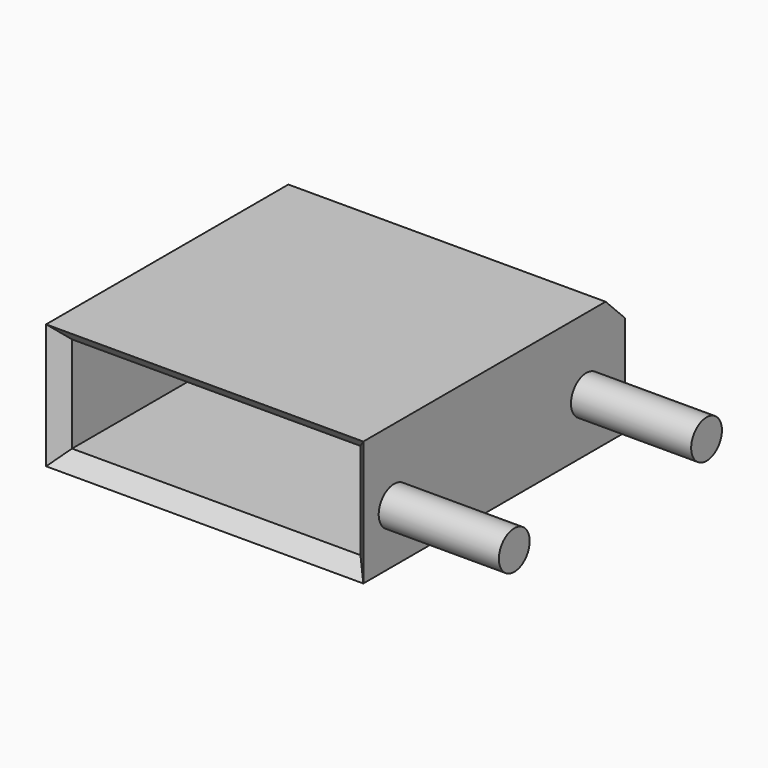
from build123d import *

# Parameters (mm, degrees)
F0_W         = 66
F0_H         = 26
F0_W_2       = 60
F0_H_2       = 20
F1_DEPTH     = 70
F2_R         = 4
F3_DEPTH     = 25
F4_T1_DEPTH  = 60
F4_T3_DEPTH  = 20
F4_T9_DEPTH  = 72.8584149398
F4_T15_DEPTH = 32.8584149398
F4_T24_DEPTH = 72.8584149398
F4_T30_DEPTH = 32.8584149398
F4_T39_DEPTH = 72.8584149398
F4_T45_DEPTH = 32.8584149398
F4_T54_DEPTH = 32.8584149398
F4_T60_DEPTH = 72.8584149398
F5_T1_DEPTH  = 91.7168298797


# Not quite as in the source:
# - a fillet or chamfer that OpenCascade refuses, or shapes differently, is made with other operations: its cross-section is extruded or revolved along the edge and cut away or added


with BuildPart() as f1:
    # F0 (on Front) → F1 (new body)
    with BuildSketch(Plane.XZ):
        with Locations((1.3007868016, 6.4724322181)):
            Rectangle(F0_W, F0_H)
        with Locations((1.3007868016, 6.4724322181)):
            Rectangle(F0_W_2, F0_H_2, mode=Mode.SUBTRACT)
    extrude(amount=F1_DEPTH)

    # F2 (on face) → F3 (join)
    with BuildSketch(Plane.YZ.offset(34.3007868016)):
        with Locations((-60, 4.4724322181)):
            Circle(F2_R)
        with Locations((-10, 4.4724322181)):
            Circle(F2_R)
    extrude(amount=F3_DEPTH)

    # F4: chamfer of 5 on 4 edges, made by hand

    # F4_s2 → F4_t1 (cut)
    with BuildSketch(Plane.YZ.offset(-28.6992131984)):
        Polygon((-70, 21.4724322181), (-65, 16.4724322181), (-70, 16.4724322181), align=None)
        Polygon((-70, -8.5275677819), (-65, -3.5275677819), (-70, -3.5275677819), align=None)
    extrude(amount=F4_T1_DEPTH, mode=Mode.SUBTRACT)

    # F4_s4 → F4_t3 (cut)
    with BuildSketch(Plane.XY.offset(-3.5275677819)):
        Polygon((-33.6992131984, -70), (-28.6992131984, -65), (-28.6992131984, -70), align=None)
        Polygon((36.3007868016, -70), (31.3007868016, -65), (31.3007868016, -70), align=None)
    extrude(amount=F4_T3_DEPTH, mode=Mode.SUBTRACT)


with BuildPart() as f4_tool7:
    # F4_s8 → F4_t9 (new body)
    with BuildSketch(Plane.YZ.offset(-41.5576281383)):
        Polygon((-70, 21.4724322181), (-65, 16.4724322181), (-70, 16.4724322181), align=None)
    extrude(amount=F4_T9_DEPTH)

    split(bisect_by=Plane.YZ.offset(-31.6992131984), keep=Keep.TOP)

    split(bisect_by=Plane.XY.offset(19.4724322181), keep=Keep.BOTTOM)

    split(bisect_by=Plane.YZ.offset(-28.6992131984), keep=Keep.BOTTOM)


with BuildPart() as f4_tool13:
    # F4_s14 → F4_t15 (new body)
    with BuildSketch(Plane.XY.offset(-3.5275677819)):
        Polygon((-33.6992131984, -70), (-28.6992131984, -65), (-28.6992131984, -70), align=None)
    extrude(amount=F4_T15_DEPTH)

    split(bisect_by=Plane.YZ.offset(-31.6992131984), keep=Keep.TOP)

    split(bisect_by=Plane.XY.offset(19.4724322181), keep=Keep.BOTTOM)

    split(bisect_by=Plane.XY.offset(16.4724322181), keep=Keep.TOP)


with BuildPart() as f4_tool7_1:
    add(f4_tool7.part)

    # F4_t19: intersect F4_tool13
    add(f4_tool13.part, mode=Mode.INTERSECT)


with BuildPart() as f1_1:
    add(f1.part)

    # F4_t5: cut F4_tool7
    add(f4_tool7_1.part, mode=Mode.SUBTRACT)


with BuildPart() as f4_tool22:
    # F4_s23 → F4_t24 (new body)
    with BuildSketch(Plane.YZ.offset(-28.6992131984)):
        Polygon((-70, 21.4724322181), (-65, 16.4724322181), (-70, 16.4724322181), align=None)
    extrude(amount=F4_T24_DEPTH)

    split(bisect_by=Plane.YZ.offset(34.3007868016), keep=Keep.BOTTOM)

    split(bisect_by=Plane.XY.offset(19.4724322181), keep=Keep.BOTTOM)

    split(bisect_by=Plane.YZ.offset(31.3007868016), keep=Keep.TOP)


with BuildPart() as f4_tool28:
    # F4_s29 → F4_t30 (new body)
    with BuildSketch(Plane.XY.offset(29.3308471579)):
        Polygon((36.3007868016, -70), (31.3007868016, -65), (31.3007868016, -70), align=None)
    extrude(amount=-F4_T30_DEPTH)

    split(bisect_by=Plane.YZ.offset(34.3007868016), keep=Keep.BOTTOM)

    split(bisect_by=Plane.XY.offset(19.4724322181), keep=Keep.BOTTOM)

    split(bisect_by=Plane.XY.offset(16.4724322181), keep=Keep.TOP)


with BuildPart() as f4_tool22_1:
    add(f4_tool22.part)

    # F4_t34: intersect F4_tool28
    add(f4_tool28.part, mode=Mode.INTERSECT)


with BuildPart() as f1_2:
    add(f1_1.part)

    # F4_t20: cut F4_tool22
    add(f4_tool22_1.part, mode=Mode.SUBTRACT)


with BuildPart() as f4_tool37:
    # F4_s38 → F4_t39 (new body)
    with BuildSketch(Plane.YZ.offset(31.3007868016)):
        Polygon((-70, -8.5275677819), (-65, -3.5275677819), (-70, -3.5275677819), align=None)
    extrude(amount=-F4_T39_DEPTH)

    split(bisect_by=Plane.XY.offset(-6.5275677819), keep=Keep.TOP)

    split(bisect_by=Plane.YZ.offset(-31.6992131984), keep=Keep.TOP)

    split(bisect_by=Plane.YZ.offset(-28.6992131984), keep=Keep.BOTTOM)


with BuildPart() as f4_tool43:
    # F4_s44 → F4_t45 (new body)
    with BuildSketch(Plane.XY.offset(-16.3859827218)):
        Polygon((-33.6992131984, -70), (-28.6992131984, -65), (-28.6992131984, -70), align=None)
    extrude(amount=F4_T45_DEPTH)

    split(bisect_by=Plane.XY.offset(-6.5275677819), keep=Keep.TOP)

    split(bisect_by=Plane.YZ.offset(-31.6992131984), keep=Keep.TOP)

    split(bisect_by=Plane.XY.offset(-3.5275677819), keep=Keep.BOTTOM)


with BuildPart() as f4_tool37_1:
    add(f4_tool37.part)

    # F4_t49: intersect F4_tool43
    add(f4_tool43.part, mode=Mode.INTERSECT)


with BuildPart() as f1_3:
    add(f1_2.part)

    # F4_t35: cut F4_tool37
    add(f4_tool37_1.part, mode=Mode.SUBTRACT)


with BuildPart() as f4_tool52:
    # F4_s53 → F4_t54 (new body)
    with BuildSketch(Plane.XY.offset(16.4724322181)):
        Polygon((36.3007868016, -70), (31.3007868016, -65), (31.3007868016, -70), align=None)
    extrude(amount=-F4_T54_DEPTH)

    split(bisect_by=Plane.XY.offset(-6.5275677819), keep=Keep.TOP)

    split(bisect_by=Plane.YZ.offset(34.3007868016), keep=Keep.BOTTOM)

    split(bisect_by=Plane.XY.offset(-3.5275677819), keep=Keep.BOTTOM)


with BuildPart() as f4_tool58:
    # F4_s59 → F4_t60 (new body)
    with BuildSketch(Plane.YZ.offset(44.1592017414)):
        Polygon((-70, -8.5275677819), (-65, -3.5275677819), (-70, -3.5275677819), align=None)
    extrude(amount=-F4_T60_DEPTH)

    split(bisect_by=Plane.XY.offset(-6.5275677819), keep=Keep.TOP)

    split(bisect_by=Plane.YZ.offset(34.3007868016), keep=Keep.BOTTOM)

    split(bisect_by=Plane.YZ.offset(31.3007868016), keep=Keep.TOP)


with BuildPart() as f4_tool52_1:
    add(f4_tool52.part)

    # F4_t64: intersect F4_tool58
    add(f4_tool58.part, mode=Mode.INTERSECT)


with BuildPart() as f1_4:
    add(f1_3.part)

    # F4_t50: cut F4_tool52
    add(f4_tool52_1.part, mode=Mode.SUBTRACT)

    # F5: chamfer of 5 on 1 edges, made by hand

    # F5_s2 → F5_t1 (cut)
    with BuildSketch(Plane.YZ.offset(-44.5576281383)):
        Polygon((-5, 19.4724322181), (0, 14.4724322181), (0, 19.4724322181), align=None)
    extrude(amount=F5_T1_DEPTH, mode=Mode.SUBTRACT)


solid = f1_4.part
